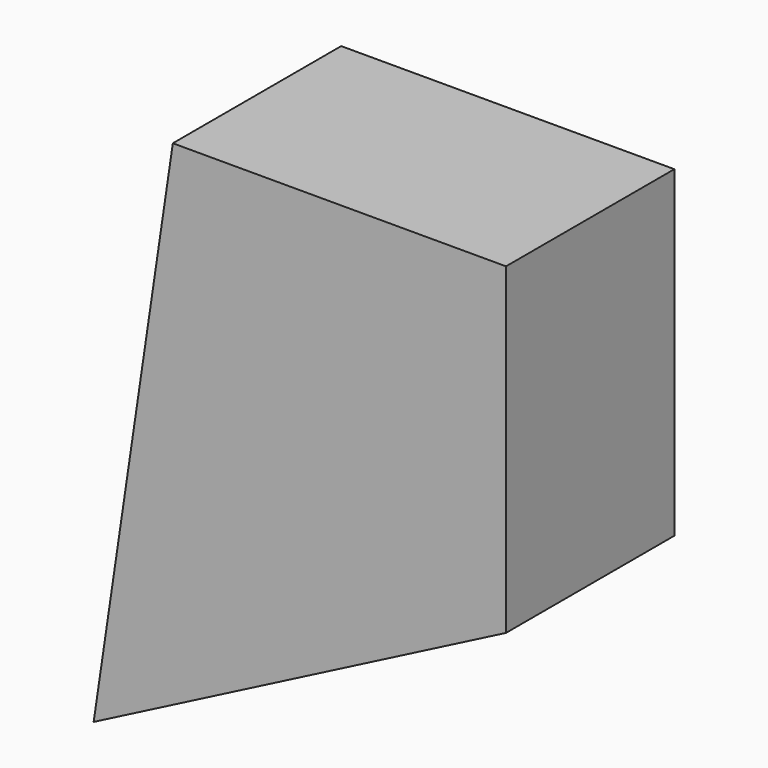
from build123d import *

# Parameters (mm, degrees)
F1_DEPTH = 25.4


# Not quite as in the source:
# - the program builds the solid bodies; features that only make, move or delete a surface that nothing else refers to are left out


with BuildPart() as f1:
    # F0 (on Front) → F1 (new body)
    with BuildSketch(Plane.XZ):
        Polygon((40.2166396379, 38.9555729926), (0, 38.9555729926), (-9.5569342375, -25.6445333362), (40.2166396379, 0), align=None)
    extrude(amount=F1_DEPTH)


solid = f1.part
